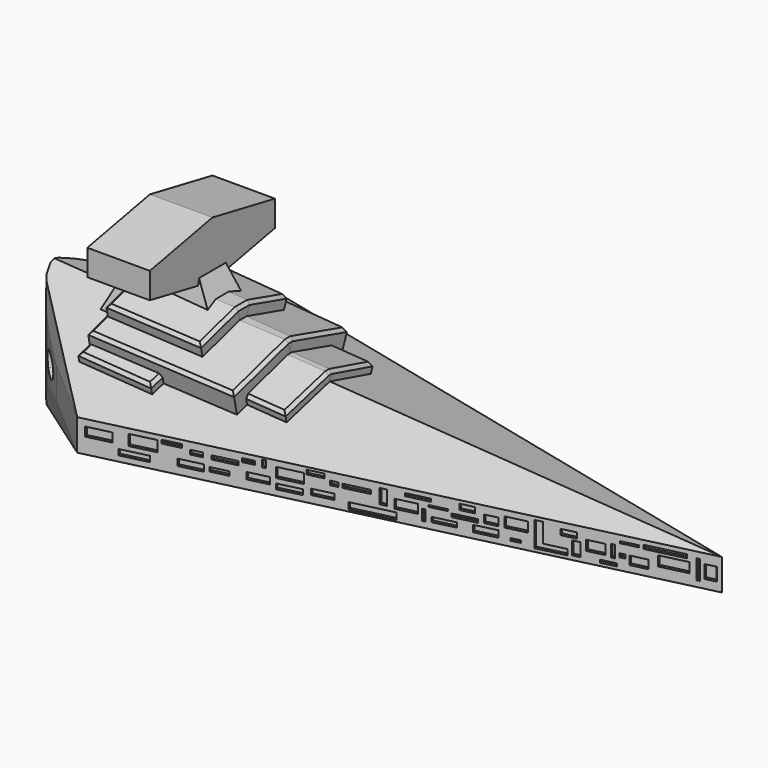
from build123d import *

# Parameters (mm, degrees)
F1_DEPTH     = 5
F6_T1_DEPTH  = 266.6511178274
F7_SIZE      = 5
F8_SIZE      = 5
F9_SIZE      = 5
F10_SIZE     = 5
F11_SIZE     = 5
F12_T1_DEPTH = 35.9996543964
F13_R        = 7.1994455106
F13_R_2      = 3.4704970512
F13_R_3      = 3.9176746903
F14_DEPTH    = 99.65128
F16_W        = 6.8071749993
F16_H        = 1.9555875333
F16_W_2      = 4.3856026605
F16_H_2      = 1.5042979503
F16_W_3      = 7.8901341185
F16_H_3      = 2.030802425
F16_W_4      = 6.03363337
F16_H_4      = 1.0530087166
F16_W_5      = 5.7242149487
F16_H_5      = 1.2034383835
F16_W_6      = 6.8071745336
F16_H_6      = 2.6325215586
F16_W_7      = 5.5695045739
F16_W_8      = 2.3206304759
F16_H_7      = 1.3538682833
F17_DEPTH    = 0.5
F18_W        = 4.3318420649
F18_H        = 1.6547280829
F18_W_2      = 5.2600950003
F18_H_2      = 2.2564470419
F18_W_3      = 5.4148025811
F18_H_3      = 1.5042980667
F18_W_4      = 4.9506761134
F18_H_4      = 1.5042981831
F18_W_5      = 6.1883404851
F18_H_5      = 2.030802425
F18_W_6      = 6.033629179
F18_H_6      = 1.8051577499
F18_W_7      = 9.2825107276
F18_H_7      = 2.1060170839
F18_W_8      = 2.939466387
F18_W_9      = 5.1053836942
F18_H_8      = 2.4820917752
F19_DEPTH    = 0.5
F23_W        = 5.7242140174
F23_H        = 1.9555875333
F23_W_2      = 4.1771307588
F23_H_2      = 3.5351002589
F23_W_3      = 7.4260160327
F23_H_3      = 1.3538682833
F23_W_4      = 3.7130117416
F23_H_4      = 1.7675501294
F23_W_5      = 4.7959685326
F23_H_5      = 1.0530086001
F23_W_6      = 6.3430517912
F23_H_6      = 2.1060173167
F23_W_7      = 3.0941665173
F23_H_7      = 1.8803725252
F23_W_8      = 5.2600950003
F23_H_8      = 1.8051577499
F23_W_9      = 4.9506723881
F23_H_9      = 1.2034383835
F23_W_10     = 2.7847513556
F23_H_10     = 1.7299427418
F24_DEPTH    = 0.5
F25_W        = 3.2488852739
F25_H        = 2.030802425
F25_W_2      = 3.5583004355
F25_H_2      = 1.0530084837
F25_W_3      = 3.8677155972
F25_H_3      = 1.3538682833
F25_W_4      = 7.1165934205
F25_H_4      = 0.7521490334
F25_W_5      = 4.7959536314
F25_H_5      = 1.579512842
F25_W_6      = 6.1883479357
F25_H_6      = 2.1812322084
F25_W_7      = 4.6412721276
F25_H_7      = 1.6547277337
F25_H_8      = 1.5042980667
F25_W_8      = 5.4147988558
F25_H_9      = 1.9555874169
F25_W_9      = 2.9394626617
F25_H_10     = 3.9111749502
F25_W_10     = 1.2376755476
F25_H_11     = 4.9641837832
F25_W_11     = 1.0829567909
F25_W_12     = 4.3318420649
F25_H_12     = 1.0530086001
F25_W_13     = 3.8677304983
F25_H_13     = 0.9025787003
F25_W_14     = 2.0111948252
F25_H_14     = 2.9333811253
F26_DEPTH    = 0.5
F28_DEPTH    = 3
F29_SIZE     = 1
F31_W        = 46.0713699278
F31_H        = 22.5975452367
F32_DEPTH    = 7
F33_SIZE     = 1
F35_W        = 29.852832627
F35_H        = 15.5214233749
F36_DEPTH    = 4
F37_SIZE     = 1
F42_W        = 14.3484091386
F42_H        = 8.7151173502
F41_W        = 46.2565384805
F41_H        = 19.8458600789
F47_DEPTH    = 10
F48_DEPTH    = 20
F49_DEPTH    = 1
F15_W        = 7.5335321017
F15_H        = 2.8581663501
F15_W_2      = 8.6636776105
F15_H_2      = 1.8051578663
F15_W_3      = 8.0448444933
F15_H_3      = 3.4598854836
F15_W_4      = 7.4260085821
F15_H_4      = 2.1060174331
F15_W_5      = 7.4260123074
F15_H_5      = 1.2034382671
F15_W_6      = 6.4977630973
F15_H_6      = 2.1060172003
F15_W_7      = 7.7354311943
F15_H_7      = 3.159025684
F15_W_8      = 6.4977481961
F15_H_8      = 1.8051576335
F15_W_9      = 13.3049190044
F15_W_10     = 6.4977556467
F15_W_11     = 7.1166008711
F15_H_9      = 1.5042980667
F15_W_12     = 4.3318271637
F15_H_10     = 1.8051574007
F15_W_13     = 7.1166157722
F15_W_14     = 6.8071931601
F15_W_15     = 4.641264677
F15_W_16     = 5.2601099014
F15_H_11     = 2.7077365667
F15_H_12     = 0.6017191336
F15_W_17     = 8.663713932
F15_W_18     = 5.6517273188
F15_H_13     = 1.0915431194
F15_W_19     = 3.534629941
F15_H_14     = 1.3537486084
F15_W_20     = 5.5739954114
F15_H_15     = 1.3002285268
F15_W_21     = 3.6123618484
F15_H_16     = 1.1450615712
F15_W_22     = 1.184374094
F15_H_17     = 2.24199472
F15_W_23     = 7.4579119682
F15_H_18     = 1.6640732065
F15_W_24     = 2.0652711391
F15_H_19     = 4.6211085282
F15_W_25     = 5.0447285175
F15_H_20     = 1.3657785021
F15_W_26     = 5.3556412458
F15_H_21     = 0.5310445558
F15_W_27     = 7.2395503521
F15_H_22     = 0.8948920295
F15_W_28     = 1.0141283274
F15_H_23     = 3.4627902787
F15_W_29     = 4.0594041348
F15_H_24     = 2.4456102401
F15_W_30     = 2.3280084133
F15_H_25     = 1.3024990913
F15_W_31     = 2.8134435415
F15_H_26     = 0.7510422729
F15_W_32     = 2.3802220821
F15_H_27     = 4.2347782291
F15_W_33     = 4.6943128109
F15_H_28     = 0.883447472
F15_W_34     = 1.2114346027
F15_H_29     = 3.8879711647
F15_W_35     = 1.6657412052
F15_H_30     = 1.1779301567
F15_W_36     = 0.9443461895
F15_H_31     = 6.2120719813
F15_W_37     = 12.0068490505
F15_H_32     = 1.1805938557
F15_W_38     = 3.5075843334
F15_H_33     = 4.1976656939
F15_W_39     = 7.2850584984
F15_H_34     = 1.0494164308
F50_DEPTH    = 1


# Not quite as in the source:
# - a fillet or chamfer that OpenCascade refuses, or shapes differently, is made with other operations: its cross-section is extruded or revolved along the edge and cut away or added
# - after a boolean that leaves OpenCascade's solid faulty, fix() repairs it
# - a feature names something its author has since deleted; it is built from what else it names


with BuildPart() as f1:
    # F0 (on Top) → F1 (new body)
    with BuildSketch(Plane.XY):
        Polygon((-48.0396403135, 0), (0, -41.5264127821), (172.8826105814, 0), (0, 41.5264127821), align=None)
    extrude(amount=F1_DEPTH)

    # F1_face (on face) → F4 section 0
    with BuildSketch(Plane(origin=(41.6143234226, 0, 5), x_dir=(1, 0, 0), z_dir=(0, 0, 1)), mode=Mode.PRIVATE) as f4_s0:
        Polygon((-89.6539637362, 0), (-41.6143234226, -41.5264127821), (131.2682871588, 0), (-41.6143234226, 41.5264127821), align=None)
    loft([Vertex(-45.1525375247, 0, 20), f4_s0.sketch])

    # F5: F1 across plane


with BuildPart() as f1_1:
    add(f1.part)
    add(f1.part.mirror(Plane.XY))

    # F6: chamfer of 10 on 1 edges, made by hand

    # F6_s2 → F6_t1 (cut)
    with BuildSketch(Plane.XY.offset(-133.3255589137)):
        Polygon((-40.4743426264, -6.5395925641), (-40.4743426264, 6.5395925641), (-48.0396403135, 0), align=None)
    extrude(amount=F6_T1_DEPTH, mode=Mode.SUBTRACT)

    # F7
    f7_edges = [f1_1.edges().sort_by_distance(p)[0] for p in [
        (-40.474343, -6.539593, 0),
    ]]
    chamfer(f7_edges, length=F7_SIZE)

    # F8
    f8_edges = [f1_1.edges().sort_by_distance(p)[0] for p in [
        (-40.474343, 6.539593, 0),
    ]]
    chamfer(f8_edges, length=F8_SIZE)

    # F9
    f9_edges = [f1_1.edges().sort_by_distance(p)[0] for p in [
        (-36.691694, 9.809389, 0),
        (-36.691694, -9.809389, 0),
    ]]
    chamfer(f9_edges, length=F9_SIZE)

    # F10
    f10_edges = [f1_1.edges().sort_by_distance(p)[0] for p in [
        (-32.909045, 13.079185, 0),
        (-32.909045, -13.079185, 0),
    ]]
    chamfer(f10_edges, length=F10_SIZE)

    # F11
    f11_edges = [f1_1.edges().sort_by_distance(p)[0] for p in [
        (-29.126396, 16.348981, 0),
        (-29.126396, -16.348981, 0),
    ]]
    chamfer(f11_edges, length=F11_SIZE)

    # F12: chamfer of 5 on 2 edges, made by hand

    # F12_s2 → F12_t1 (cut)
    with BuildSketch(Plane.XY.offset(-17.9998271982)):
        Polygon((-28.9457019516, 16.1509365277), (-21.5610984085, 22.8885739743), (-25.3437472521, 19.6187776923), align=None)
        Polygon((-21.5610984085, -22.8885739743), (-28.9457019516, -16.1509365277), (-25.3437472521, -19.6187776923), align=None)
    extrude(amount=F12_T1_DEPTH, mode=Mode.SUBTRACT)

    # F13 (on Right) → F14 (cut)
    with BuildSketch(Plane.YZ):
        Circle(F13_R)
        with Locations((16.0207748413, 0)):
            Circle(F13_R_2)
        with Locations((-16.6224949062, 0)):
            Circle(F13_R_3)
    extrude(amount=-F14_DEPTH, mode=Mode.SUBTRACT)

    # F16 (on face) → F17 (cut)
    with BuildSketch(Plane(origin=(9.4305415291, 39.2611961766, 0), x_dir=(-0.9723431416, 0.2335568773, 0), z_dir=(0.2335568773, 0.9723431416, 0))):
        with Locations((4.5403081458, 2.4068769417)):
            Rectangle(F16_W, F16_H)
        with Locations((2.1928013302, -2.1812321502)):
            Rectangle(F16_W_2, F16_H_2)
        with Locations((-6.830770988, 1.0154012125)):
            Rectangle(F16_W_3, F16_H_3)
        with Locations((-6.3666456845, -2.8581663501)):
            Rectangle(F16_W_4, F16_H_4)
        with Locations((-17.5056620501, 2.482091717)):
            Rectangle(F16_W_5, F16_H_5)
        with Locations((-16.3453463465, -1.3162607793)):
            Rectangle(F16_W_6, F16_H_6)
        with Locations((-28.1805498526, 1.0154012125)):
            Rectangle(F16_W_7, F16_H_3)
        with Locations((-23.3072331175, -3.0085961334)):
            Rectangle(F16_W_8, F16_H_7)
    extrude(amount=-F17_DEPTH, mode=Mode.SUBTRACT)

    # F18 (on face) → F19 (cut)
    with BuildSketch(Plane(origin=(9.4305415291, 39.2611961766, 0), x_dir=(-0.9723431416, 0.2335568773, 0), z_dir=(0.2335568773, 0.9723431416, 0))):
        with Locations((-29.0314480662, -2.4068768835)):
            Rectangle(F18_W, F18_H)
        with Locations((-36.6121679544, -1.5042980376)):
            Rectangle(F18_W_2, F18_H_2)
        with Locations((-37.6177746803, 2.3316618754)):
            Rectangle(F18_W_3, F18_H_3)
        with Locations((-43.4193443507, -2.6325216168)):
            Rectangle(F18_W_4, F18_H_4)
        with Locations((-46.5135164559, 1.0154012125)):
            Rectangle(F18_W_5, F18_H_5)
        with Locations((-53.3980466425, -2.7829514001)):
            Rectangle(F18_W_6, F18_H_6)
        with Locations((-56.1054479331, 2.482091717)):
            Rectangle(F18_W_7, F18_H_7)
        with Locations((-60.9787646681, -2.33166205)):
            Rectangle(F18_W_8, F18_H_6)
        with Locations((-67.4765221775, 1.2410458876)):
            Rectangle(F18_W_9, F18_H_8)
    extrude(amount=-F19_DEPTH, mode=Mode.SUBTRACT)

    # F21 (on offset) → F22 (revolve)
    with BuildSketch(Plane.XY.offset(-10)):
        with BuildLine():
            Line((0, -12.0547582723), (0, 12.0547582723))
            ThreePointArc((0, 12.0547582723), (-12.0547582723, 0), (0, -12.0547582723))
        make_face()
    revolve(axis=Axis((0, 0, -10), (0, -1, 0)))

    # F23 (on face) → F24 (cut)
    with BuildSketch(Plane(origin=(9.4305415291, 39.2611961766, 0), x_dir=(-0.9723431416, 0.2335568773, 0), z_dir=(0.2335568773, 0.9723431416, 0))):
        with Locations((-67.1671070158, -2.4068769417)):
            Rectangle(F23_W, F23_H)
        with Locations((-73.9742852747, 1.7675501294)):
            Rectangle(F23_W_2, F23_H_2)
        with Locations((-77.4552263319, -3.0085961334)):
            Rectangle(F23_W_3, F23_H_3)
        with Locations((-79.3117284775, 0.8837750647)):
            Rectangle(F23_W_4, F23_H_4)
        with Locations((-85.4227170348, -2.4068768253)):
            Rectangle(F23_W_5, F23_H_5)
        with Locations((-86.1962586641, 2.7829514001)):
            Rectangle(F23_W_6, F23_H_6)
        with Locations((-94.0090417862, -0.9401862626)):
            Rectangle(F23_W_7, F23_H_7)
        with Locations((-101.7444729805, -2.7829514001)):
            Rectangle(F23_W_8, F23_H_8)
        with Locations((-93.390211463, 2.3316619336)):
            Rectangle(F23_W_9, F23_H_9)
        with Locations((-101.2803427875, 0.8649713709)):
            Rectangle(F23_W_10, F23_H_10)
    extrude(amount=-F24_DEPTH, mode=Mode.SUBTRACT)

    # F25 (on face) → F26 (cut)
    with BuildSketch(Plane(origin=(9.4305415291, 39.2611961766, 0), x_dir=(-0.9723431416, 0.2335568773, 0), z_dir=(0.2335568773, 0.9723431416, 0))):
        with Locations((-106.3083708286, 1.0154012125)):
            Rectangle(F25_W, F25_H)
        with Locations((-108.0101691186, -3.008596017)):
            Rectangle(F25_W_2, F25_H_2)
        with Locations((-111.2590506673, 2.7077365667)):
            Rectangle(F25_W_3, F25_H_3)
        with Locations((-115.8229522407, -2.2564470419)):
            Rectangle(F25_W_4, F25_H_4)
        with Locations((-117.6020950079, 0.789756421)):
            Rectangle(F25_W_5, F25_H_5)
        with Locations((-126.9619688392, -1.0906161042)):
            Rectangle(F25_W_6, F25_H_6)
        with Locations((-124.1772137582, 2.2564470419)):
            Rectangle(F25_W_7, F25_H_7)
        with Locations((-134.6200406551, -2.9333812417)):
            Rectangle(F25_W_3, F25_H_8)
        with Locations((-132.7635422349, 2.5573065504)):
            Rectangle(F25_W_8, F25_H_9)
        with Locations((-140.0348395109, -0.2256447333)):
            Rectangle(F25_W_9, F25_H_10)
        with Locations((-147.2287848592, 0.3008596832)):
            Rectangle(F25_W_10, F25_H_11)
        with Locations((-143.5931324959, -0.789756421)):
            Rectangle(F25_W_11, F25_H_5)
        with Locations((-152.4888798594, 1.9555874751)):
            Rectangle(F25_W_12, F25_H_12)
        Polygon((-154.190659523, -2.1812322084), (-154.190659523, -3.0838109087), (-150.322958827, -3.0838109087), (-150.322958827, 0), (-154.190659523, 0), align=None)
        with Locations((-156.1245247722, -2.6325215586)):
            Rectangle(F25_W_13, F25_H_13)
        with Locations((-159.9922403693, 1.4666905627)):
            Rectangle(F25_W_14, F25_H_14)
    extrude(amount=-F26_DEPTH, mode=Mode.SUBTRACT)

    # F27 (on face) → F28 (join)
    with BuildSketch(Plane(origin=(1.0694322316, 4.4522563751, 15.5449210007), x_dir=(0.9978200953, -0.0181705694, -0.0634420038), z_dir=(0.065992859, 0.2747412306, 0.9592508529))):
        Polygon((-13.0104542618, 21.9520504423), (-12.503531557, -4.8676025547), (46.5383879441, -3.7516414521), (46.2077463527, 13.7415437322), (10.5043951413, 13.0667087756), (10.3281140279, 22.3931765883), align=None)
    extrude(amount=F28_DEPTH)

    # F29
    f29_edges = [f1_1.edges().sort_by_distance(p)[0] for p in [
        (-11.461773, 13.720319, 16.879974),
        (-0.070836, 26.616414, 12.402721),
        (11.660959, 22.131829, 12.880057),
        (29.561668, 17.647244, 12.932996),
        (47.539389, 9.235734, 14.105356),
    ]]
    chamfer(f29_edges, length=F29_SIZE)

    # F30: F1 across plane


with BuildPart() as f1_2:
    add(f1_1.part)
    add(f1_1.part.mirror(Plane.XZ))

    # F31 (on face) → F32 (join)
    with BuildSketch(Plane(origin=(1.0694322316, 4.4522563751, 15.5449210007), x_dir=(0.9978200953, -0.0181705694, -0.0634420038), z_dir=(0.065992859, 0.2747412306, 0.9592508529))):
        with Locations((10.5321534069, 6.4311700636)):
            Rectangle(F31_W, F31_H)
    extrude(amount=F32_DEPTH)

    # F33
    f33_edges = [f1_2.edges().sort_by_distance(p)[0] for p in [
        (-10.944893, 12.785224, 21.282158),
        (12.040577, 23.228688, 16.709708),
        (35.026046, 11.948081, 18.359298),
    ]]
    chamfer(f33_edges, length=F33_SIZE)

    # F34: F1 across plane


with BuildPart() as f1_3:
    add(f1_2.part)
    add(f1_2.part.mirror(Plane.XZ))

    # F35 (on face) → F36 (join)
    with BuildSketch(Plane(origin=(1.5313822449, 6.3754449892, 22.259676971), x_dir=(0.9978200953, -0.0181705694, -0.0634420038), z_dir=(0.065992859, 0.2747412306, 0.9592508529))):
        with Locations((3.4228847565, 2.8931091327)):
            Rectangle(F35_W, F35_H)
    extrude(amount=F36_DEPTH)

    # F37
    f37_edges = [f1_3.edges().sort_by_distance(p)[0] for p in [
        (-9.683101, 10.464716, 26.029895),
        (5.210777, 17.654227, 22.946087),
        (20.104655, 9.922273, 24.135971),
    ]]
    chamfer(f37_edges, length=F37_SIZE)

    # F38: F1 across plane


with BuildPart() as f1_4:
    add(f1_3.part)
    add(f1_3.part.mirror(Plane.XZ))

    # F42 (on offset) → F43 section 0
    with BuildSketch(Plane.XY.offset(38)):
        Rectangle(F42_W, F42_H)
    # F41 (on offset) → F43 section 1
    with BuildSketch(Plane.XY.offset(8)):
        Rectangle(F41_W, F41_H)
    loft()

    # F36_face (on face) → F44 section 0
    with BuildSketch(Plane(origin=(23.5236257865, 0.9376230945, 20.952106045), x_dir=(1, 0, 0), z_dir=(0, -0.9613464967, 0.2753414487))):
        with BuildLine():
            Line((-3.4849636224, 4.5368239341), (-4.4167908587, 5.6006368884))
            Line((-4.4167908587, 5.6006368884), (-10.3471371068, 5.9928523848))
            add(Edge.make_bspline(
                [(-10.3471371068, 5.9928523848), (-9.6838277139, 4.6954159018), (-9.0104054574, 3.3781986071), (-8.3285445082, 2.0444751874), (-7.6397158256, 0.6971228465), (-6.9451420434, -0.661466938), (-6.2457887493, -2.0294054718), (-5.5423626746, -3.4053103844)],
                knots=[0, 0, 0, 0, 0, 0, 0, 0, 0.8277080088, 0.8277080088, 0.8277080088, 0.8277080088, 0.8277080088, 0.8277080088, 0.8277080088, 0.8277080088], degree=7))
            Line((-5.5423626746, -3.4053103844), (11.2415519286, -3.4053103844))
            Line((11.2415519286, -3.4053103844), (11.4364272811, -0.4587712339))
            Line((11.4364272811, -0.4587712339), (10.5046000448, 0.6050417205))
            Line((10.5046000448, 0.6050417205), (-3.6829421995, 1.5433636482))
            Line((-3.6829421995, 1.5433636482), (-3.4849636224, 4.5368239341))
        make_face()
    # F38_face (on face) → F44 section 1
    with BuildSketch(Plane(origin=(23.5236257865, -0.9376230945, 20.952106045), x_dir=(-1, 0, 0), z_dir=(0, 0.9613464967, 0.2753414487))):
        with BuildLine():
            Line((-11.4364272811, -0.4587712339), (-11.2415519286, -3.4053103844))
            Line((-11.2415519286, -3.4053103844), (5.5423626746, -3.4053103844))
            add(Edge.make_bspline(
                [(5.5423626746, -3.4053103844), (6.2457887488, -2.0294054726), (6.9451420418, -0.6614669412), (7.6397158237, 0.6971228428), (8.3285445074, 2.0444751858), (9.0104054585, 3.3781986093), (9.683827716, 4.6954159059), (10.3471371068, 5.9928523848)],
                knots=[0.1722919911, 0.1722919911, 0.1722919911, 0.1722919911, 0.1722919911, 0.1722919911, 0.1722919911, 0.1722919911, 1, 1, 1, 1, 1, 1, 1, 1], degree=7))
            Line((10.3471371068, 5.9928523848), (4.4167908587, 5.6006368884))
            Line((4.4167908587, 5.6006368884), (3.4849636224, 4.5368239341))
            Line((3.4849636224, 4.5368239341), (3.6829421995, 1.5433636482))
            Line((3.6829421995, 1.5433636482), (-10.5046000448, 0.6050417205))
            Line((-10.5046000448, 0.6050417205), (-11.4364272811, -0.4587712339))
        make_face()
    loft()

    add(f1_4.part.fix(), mode=Mode.REPLACE)

    # F30_face (on face) → F45 section 0
    with BuildSketch(Plane(origin=(41.0533298317, -0.4079402799, 15.5004123562), x_dir=(-0.9998077545, 0.0196075017, 0), z_dir=(0.0188565949, 0.9615182038, 0.2740933648))):
        Polygon((-6.4438018347, -1.9496636488), (6.4959850819, -1.0238270094), (6.2818835978, 1.9685233302), (-5.6604532055, 1.1140538521), (-6.5865361574, 0.0452365776), align=None)
    # F28_face (on face) → F45 section 1
    with BuildSketch(Plane(origin=(41.0533298317, 0.4079402799, 15.5004123562), x_dir=(0.9998077545, 0.0196075017, 0), z_dir=(0.0188565949, -0.9615182038, 0.2740933648))):
        Polygon((-6.4959850819, -1.0238270094), (6.4438018347, -1.9496636488), (6.5865361574, 0.0452365776), (5.6604532055, 1.1140538521), (-6.2818835978, 1.9685233302), align=None)
    loft()

    add(f1_4.part.fix(), mode=Mode.REPLACE)

    # F46 (on Right) → F47 (join)
    with BuildSketch(Plane.YZ):
        Polygon((25, 34.4237024674), (25, 42.7191503362), (0, 47.5714264018), (-25, 42.7191503362), (-25, 34.4237024674), (0, 29.5714264018), align=None)
    extrude(amount=F47_DEPTH)

    # F48 (add): a face of the model
    f48_faces = [f1_4.faces().sort_by_distance(p)[0] for p in [
        (10, -2e-10, 38.8980351821),
    ]]
    extrude(f48_faces, amount=-F48_DEPTH)

    # F16 (on face) + F18 (on face) + F23 (on face) + F25 (on face) → F49 (cut)
    with BuildSketch(Plane(origin=(9.4305415291, 39.2611961766, 0), x_dir=(-0.9723431416, 0.2335568773, 0), z_dir=(0.2335568773, 0.9723431416, 0))):
        with Locations((4.5403081458, 2.4068769417)):
            Rectangle(F16_W, F16_H)
        with Locations((2.1928013302, -2.1812321502)):
            Rectangle(F16_W_2, F16_H_2)
        with Locations((-6.830770988, 1.0154012125)):
            Rectangle(F16_W_3, F16_H_3)
        with Locations((-6.3666456845, -2.8581663501)):
            Rectangle(F16_W_4, F16_H_4)
        with Locations((-17.5056620501, 2.482091717)):
            Rectangle(F16_W_5, F16_H_5)
        with Locations((-16.3453463465, -1.3162607793)):
            Rectangle(F16_W_6, F16_H_6)
        with Locations((-28.1805498526, 1.0154012125)):
            Rectangle(F16_W_7, F16_H_3)
        with Locations((-23.3072331175, -3.0085961334)):
            Rectangle(F16_W_8, F16_H_7)
    with BuildSketch(Plane(origin=(9.4305415291, 39.2611961766, 0), x_dir=(-0.9723431416, 0.2335568773, 0), z_dir=(0.2335568773, 0.9723431416, 0))):
        with Locations((-29.0314480662, -2.4068768835)):
            Rectangle(F18_W, F18_H)
        with Locations((-36.6121679544, -1.5042980376)):
            Rectangle(F18_W_2, F18_H_2)
        with Locations((-37.6177746803, 2.3316618754)):
            Rectangle(F18_W_3, F18_H_3)
        with Locations((-43.4193443507, -2.6325216168)):
            Rectangle(F18_W_4, F18_H_4)
        with Locations((-46.5135164559, 1.0154012125)):
            Rectangle(F18_W_5, F18_H_5)
        with Locations((-53.3980466425, -2.7829514001)):
            Rectangle(F18_W_6, F18_H_6)
        with Locations((-56.1054479331, 2.482091717)):
            Rectangle(F18_W_7, F18_H_7)
        with Locations((-60.9787646681, -2.33166205)):
            Rectangle(F18_W_8, F18_H_6)
        with Locations((-67.4765221775, 1.2410458876)):
            Rectangle(F18_W_9, F18_H_8)
    with BuildSketch(Plane(origin=(9.4305415291, 39.2611961766, 0), x_dir=(-0.9723431416, 0.2335568773, 0), z_dir=(0.2335568773, 0.9723431416, 0))):
        with Locations((-67.1671070158, -2.4068769417)):
            Rectangle(F23_W, F23_H)
        with Locations((-73.9742852747, 1.7675501294)):
            Rectangle(F23_W_2, F23_H_2)
        with Locations((-77.4552263319, -3.0085961334)):
            Rectangle(F23_W_3, F23_H_3)
        with Locations((-79.3117284775, 0.8837750647)):
            Rectangle(F23_W_4, F23_H_4)
        with Locations((-85.4227170348, -2.4068768253)):
            Rectangle(F23_W_5, F23_H_5)
        with Locations((-86.1962586641, 2.7829514001)):
            Rectangle(F23_W_6, F23_H_6)
        with Locations((-94.0090417862, -0.9401862626)):
            Rectangle(F23_W_7, F23_H_7)
        with Locations((-101.7444729805, -2.7829514001)):
            Rectangle(F23_W_8, F23_H_8)
        with Locations((-93.390211463, 2.3316619336)):
            Rectangle(F23_W_9, F23_H_9)
        with Locations((-101.2803427875, 0.8649713709)):
            Rectangle(F23_W_10, F23_H_10)
    with BuildSketch(Plane(origin=(9.4305415291, 39.2611961766, 0), x_dir=(-0.9723431416, 0.2335568773, 0), z_dir=(0.2335568773, 0.9723431416, 0))):
        with Locations((-106.3083708286, 1.0154012125)):
            Rectangle(F25_W, F25_H)
        with Locations((-108.0101691186, -3.008596017)):
            Rectangle(F25_W_2, F25_H_2)
        with Locations((-111.2590506673, 2.7077365667)):
            Rectangle(F25_W_3, F25_H_3)
        with Locations((-115.8229522407, -2.2564470419)):
            Rectangle(F25_W_4, F25_H_4)
        with Locations((-117.6020950079, 0.789756421)):
            Rectangle(F25_W_5, F25_H_5)
        with Locations((-126.9619688392, -1.0906161042)):
            Rectangle(F25_W_6, F25_H_6)
        with Locations((-124.1772137582, 2.2564470419)):
            Rectangle(F25_W_7, F25_H_7)
        with Locations((-134.6200406551, -2.9333812417)):
            Rectangle(F25_W_3, F25_H_8)
        with Locations((-132.7635422349, 2.5573065504)):
            Rectangle(F25_W_8, F25_H_9)
        with Locations((-140.0348395109, -0.2256447333)):
            Rectangle(F25_W_9, F25_H_10)
        with Locations((-147.2287848592, 0.3008596832)):
            Rectangle(F25_W_10, F25_H_11)
        with Locations((-143.5931324959, -0.789756421)):
            Rectangle(F25_W_11, F25_H_5)
        with Locations((-152.4888798594, 1.9555874751)):
            Rectangle(F25_W_12, F25_H_12)
        Polygon((-154.190659523, -2.1812322084), (-154.190659523, -3.0838109087), (-150.322958827, -3.0838109087), (-150.322958827, 0), (-154.190659523, 0), align=None)
        with Locations((-156.1245247722, -2.6325215586)):
            Rectangle(F25_W_13, F25_H_13)
        with Locations((-159.9922403693, 1.4666905627)):
            Rectangle(F25_W_14, F25_H_14)
    extrude(amount=-F49_DEPTH, mode=Mode.SUBTRACT)

    # F15 (on face) → F50 (cut)
    with BuildSketch(Plane(origin=(9.4305415291, -39.2611961766, 0), x_dir=(0.9723431416, 0.2335568773, 0), z_dir=(0.2335568773, -0.9723431416, 0))):
        with Locations((-3.7667660508, 1.429083175)):
            Rectangle(F15_W, F15_H)
        with Locations((5.9798737057, -2.3316619918)):
            Rectangle(F15_W_2, F15_H_2)
        with Locations((8.4552112967, 1.7299427418)):
            Rectangle(F15_W_3, F15_H_3)
        with Locations((21.6054376215, -1.579512842)):
            Rectangle(F15_W_4, F15_H_4)
        with Locations((31.0426596552, 1.8803725252)):
            Rectangle(F15_W_5, F15_H_5)
        with Locations((40.1704646647, -1.1282236082)):
            Rectangle(F15_W_6, F15_H_6)
        with Locations((48.9888526499, 1.579512842)):
            Rectangle(F15_W_7, F15_H_7)
        with Locations((57.9619519413, -1.7299427418)):
            Rectangle(F15_W_8, F15_H_8)
        with Locations((67.399173975, 1.8803725252)):
            Rectangle(F15_W_7, F15_H_5)
        with Locations((71.7310160398, -3.3846707083)):
            Rectangle(F15_W_9, F15_H_4)
        with Locations((81.0135304928, 0)):
            Rectangle(F15_W_10, F15_H)
        with Locations((91.5337055922, -2.1812322084)):
            Rectangle(F15_W_11, F15_H_9)
        with Locations((97.8767648339, 3.0838109087)):
            Rectangle(F15_W_12, F15_H_10)
        with Locations((102.9821336269, -2.1812322084)):
            Rectangle(F15_W_13, F15_H_6)
        with Locations((111.3363951445, 1.579512842)):
            Rectangle(F15_W_10, F15_H_7)
        with Locations((122.1660003066, -3.0838109087)):
            Rectangle(F15_W_14, F15_H_10)
        Polygon((118.7624037266, -3.9863896091), (118.7624037266, -2.1812322084), (118.7624037266, 3.9863896091), (116.3731068373, 3.9863896091), (116.3731068373, -3.9863896091), align=None)
        with Locations((125.8790045977, 2.1812322084)):
            Rectangle(F15_W_15, F15_H_8)
        with Locations((133.3050131798, 0)):
            Rectangle(F15_W_16, F15_H_7)
        with Locations((145.2175676823, -1.579512842)):
            Rectangle(F15_W_16, F15_H_11)
        with Locations((142.5875127316, 2.9333811253)):
            Rectangle(F15_W_16, F15_H_12)
        with Locations((154.8095047474, 0)):
            Rectangle(F15_W_17, F15_H_7)
        with Locations((16.4259560406, 3.2571696211)):
            Rectangle(F15_W_18, F15_H_13)
        with Locations((23.1713857502, 2.0522626583)):
            Rectangle(F15_W_19, F15_H_14)
        with Locations((29.5133776963, -1.5912930248)):
            Rectangle(F15_W_20, F15_H_15)
        with Locations((37.5283285975, 2.9843836091)):
            Rectangle(F15_W_21, F15_H_16)
        with Locations((41.7976565659, 3.2643205486)):
            Rectangle(F15_W_22, F15_H_17)
        with Locations((48.7984567881, -2.3379749618)):
            Rectangle(F15_W_23, F15_H_18)
        with Locations((74.7364461422, 1.2228051201)):
            Rectangle(F15_W_24, F15_H_19)
        with Locations((56.0343116522, 3.5346099176)):
            Rectangle(F15_W_25, F15_H_20)
        with Locations((89.8410305381, 1.4512954513)):
            Rectangle(F15_W_26, F15_H_21)
        with Locations((84.3095928431, 3.2046709675)):
            Rectangle(F15_W_27, F15_H_22)
        with Locations((85.8492851257, -1.429083175)):
            Rectangle(F15_W_28, F15_H_23)
        with Locations((104.5107394457, 1.2228051201)):
            Rectangle(F15_W_29, F15_H_24)
        with Locations((61.1973181367, 1.9299029373)):
            Rectangle(F15_W_30, F15_H_25)
        with Locations((111.2331673503, -2.9557719827)):
            Rectangle(F15_W_31, F15_H_26)
        with Locations((127.9059797525, -1.579512842)):
            Rectangle(F15_W_32, F15_H_27)
        with Locations((136.8455588818, -3.6372600589)):
            Rectangle(F15_W_33, F15_H_28)
        with Locations((138.0569934845, 0)):
            Rectangle(F15_W_34, F15_H_29)
        with Locations((140.70700109, -0.7660554838)):
            Rectangle(F15_W_35, F15_H_30)
        with Locations((161.5595072508, 0)):
            Rectangle(F15_W_36, F15_H_31)
        with Locations((152.453199029, 3.0592856929)):
            Rectangle(F15_W_37, F15_H_32)
        with Locations((164.999678731, -0.1545521809)):
            Rectangle(F15_W_38, F15_H_33)
        with Locations((97.2082987428, 0.2389790316)):
            Rectangle(F15_W_39, F15_H_34)
    extrude(amount=-F50_DEPTH, mode=Mode.SUBTRACT)


solid = f1_4.part
